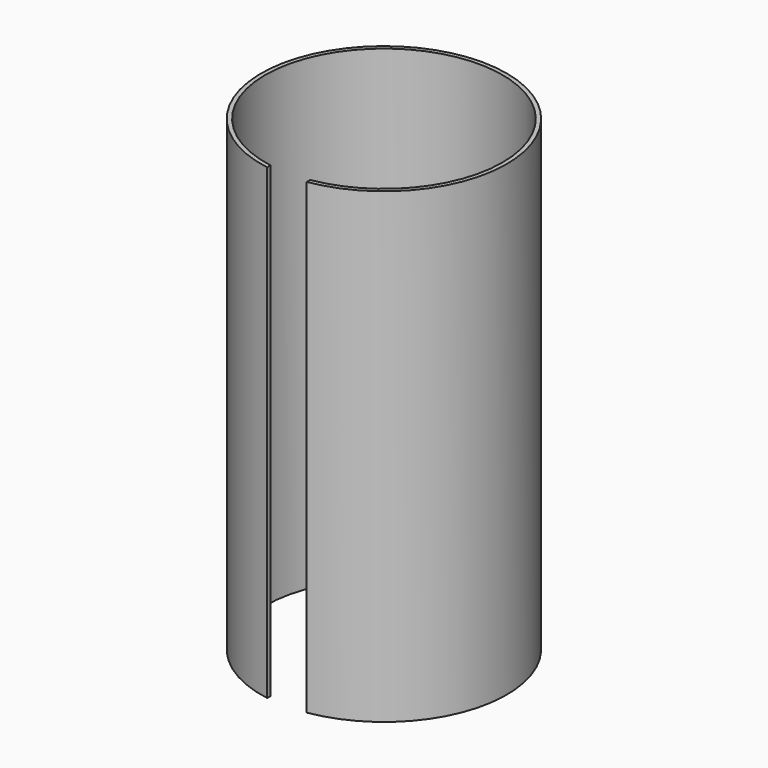
from build123d import *

# Parameters (mm, degrees)
F1_DEPTH = 39


# Not quite as in the source:
# - the program builds the solid bodies; features that only make, move or delete a surface that nothing else refers to are left out


with BuildPart() as f1:
    # F0 (on Top) → F1 (new body)
    with BuildSketch(Plane.XY):
        with BuildLine():
            Line((1.65, -9.7615316421), (1.65, -10.1163234428))
            ThreePointArc((1.65, -10.1163234428), (0, 10.25), (-1.65, -10.1163234428))
            Line((-1.65, -10.1163234428), (-1.65, -9.7615316421))
            ThreePointArc((-1.65, -9.7615316421), (0, 9.9), (1.65, -9.7615316421))
        make_face()
    extrude(amount=F1_DEPTH)


solid = f1.part
